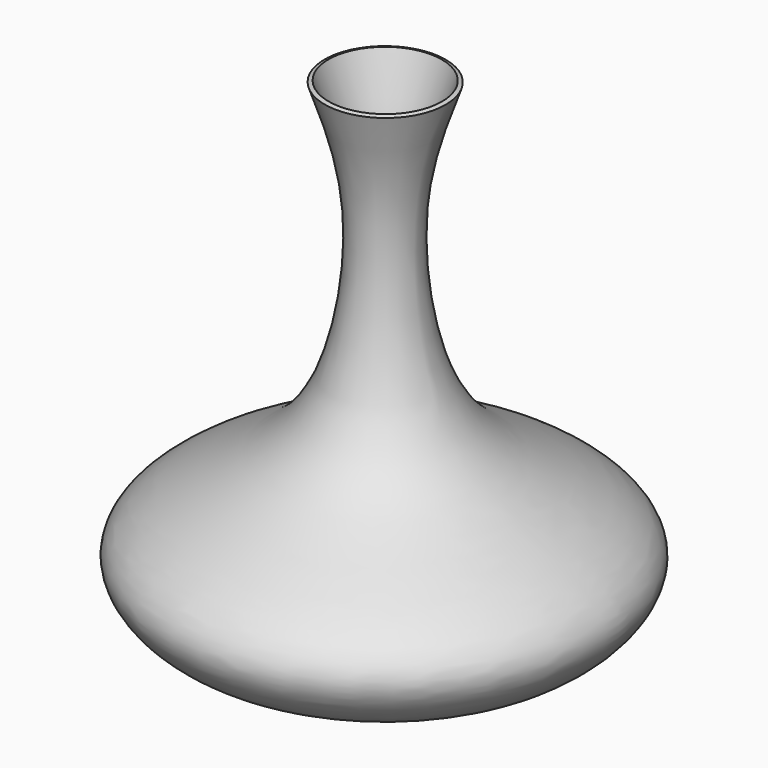
from build123d import *


# Not quite as in the source:
# - the dataset's text gives a spline's control points without its knots; the knots are read off the source's solid


with BuildPart() as f1:
    # F0 (on Front) → F1 (revolve)
    with BuildSketch(Plane.XZ):
        with BuildLine():
            add(Edge.make_bspline(
                [(18.9444348216, 63.3003115654), (15.1583460352, 52.7077048564), (6.8011243039, 29.3261182179), (15.0053171062, -27.9103205912), (46.9973189865, -44.0014512847), (76.8786921466, -62.6556225421), (47.2887007449, -91.7076474521), (17.2467797564, -81.929515972), (0, -76.3159841299)],
                knots=[0, 0, 0, 0, 0.1641683639, 0.3623769796, 0.5257360393, 0.6661432232, 0.8083360148, 1, 1, 1, 1], degree=3))
            Line((18.9444348216, 63.3003115654), (17.7485304475, 63.7277606594))
            add(Edge.make_bspline(
                [(17.7485304475, 63.7277606594), (17.0278357184, 61.7114223607), (15.5828567579, 57.6688917803), (13.5251494699, 51.4398970978), (11.7003872018, 44.911890298), (10.4776627275, 39.1135324942), (9.7403978412, 34.1947588422), (9.3229241914, 30.3510844494), (9.0573220661, 26.3309271053), (8.9179365599, 20.7566783134), (9.1500107751, 13.4914939354), (10.1035119055, 4.5943178423), (11.7584801101, -4.1794852391), (13.7470805103, -11.1376469127), (15.7217102915, -16.3427447869), (17.4001220252, -20.0278273613), (19.2823761791, -23.459322929), (21.3758414335, -26.5887556311), (23.6547132082, -29.4199602875), (26.9137998196, -32.8485357828), (31.346944767, -36.563541554), (37.0790740824, -40.3891659081), (42.0771574998, -43.2886275038), (46.1375402905, -45.5749082913), (49.2014304936, -47.3095956307), (52.2461164174, -49.088262265), (56.1685347741, -51.5198359647), (59.7320249257, -54.0504306224), (62.6192040086, -56.6720797593), (64.3695124165, -58.6726713661), (65.6360447788, -60.6896659129), (66.374498543, -62.7082018191), (66.560482684, -64.7426175743), (66.178530826, -66.9311955648), (65.2464853242, -69.2210068754), (63.7967366938, -71.54065869), (61.8807530023, -73.816601606), (59.5574217823, -75.9809020775), (56.8891128752, -77.9702473906), (53.9394543076, -79.7249536055), (51.3008228223, -80.9438635706), (49.1134916348, -81.746091379), (46.887599835, -82.4227115579), (44.025953924, -83.0363056188), (39.2852428974, -83.5638654061), (33.0737059383, -83.440354947), (25.2439527171, -82.2705970591), (17.1294499111, -80.3232236231), (8.8191465798, -77.8508195535), (3.20508103, -76.0236049621), (0.3930667288, -75.1083424005)],
                knots=[-1e-10, -1e-10, -1e-10, -1e-10, 0.0312499999, 0.0624999999, 0.0937499999, 0.1249999999, 0.1406249999, 0.1562499999, 0.1718749999, 0.1874999999, 0.2187499999, 0.2499999999, 0.2812499999, 0.3124999999, 0.3281249999, 0.3437499999, 0.3593749999, 0.3749999999, 0.3906249999, 0.4062499999, 0.4374999999, 0.46875, 0.5, 0.515625, 0.53125, 0.546875, 0.5625, 0.59375, 0.609375, 0.625, 0.640625, 0.65625, 0.671875, 0.6875, 0.703125, 0.71875, 0.734375, 0.75, 0.765625, 0.78125, 0.796875, 0.8046875, 0.8125, 0.828125, 0.84375, 0.875, 0.90625, 0.9375, 0.96875, 1, 1, 1, 1], degree=3))
            Line((0.3930667288, -75.1083424005), (0.0034004949, -75.1083424005))
            Line((0.0034004949, -75.1083424005), (0, -76.3159841299))
        make_face()
    revolve(axis=Axis((0.1965333644, 0, -6.5197050571), (0.0028158032, 0, 0.9999960356)))


solid = f1.part
